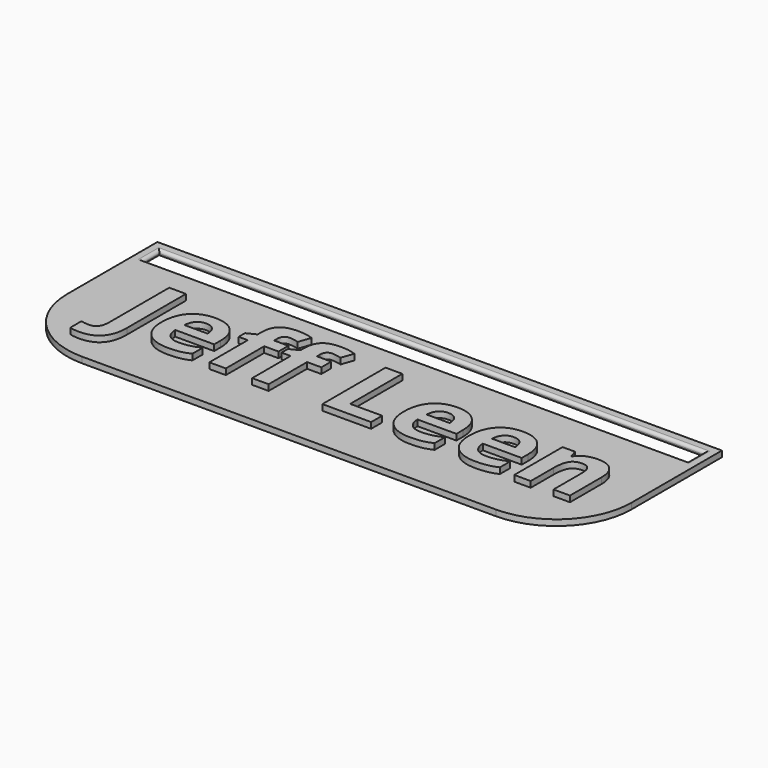
from build123d import *

# Parameters (mm, degrees)
F0_W         = 190.5
F0_H         = 63.5
F1_DEPTH     = 2
F2_W         = 183.896
F2_H         = 7.62
F3_DEPTH     = 25.4
F4_R         = 0.99999
F5_R         = 0.99999
F6_R         = 25.4
F7_TEXT_SIZE = 37.3212771969
F8_DEPTH     = 2


# Not quite as in the source:
# - a fillet or chamfer is up to 0.001 mm smaller than in the source, because OpenCascade refuses the exact size
# - Text() gives the source's letters only with a copy of the font that has no kerning and outlines rounded to 1/6400 em; it was checked with that copy


with BuildPart() as f1:
    # F0 (on Top) → F1 (new body)
    with BuildSketch(Plane.XY):
        with Locations((1.791532172, 31.75)):
            Rectangle(F0_W, F0_H)
    extrude(amount=F1_DEPTH)

    # F2 (on face) → F3 (cut)
    with BuildSketch(Plane.XY.offset(2)):
        with Locations((1.791532172, 56.388)):
            Rectangle(F2_W, F2_H)
    extrude(amount=-F3_DEPTH, mode=Mode.SUBTRACT)

    # F4 (radius 1 in the source; OpenCascade refuses exactly that, so slightly less here)
    f4_edges = [f1.edges().sort_by_distance(p)[0] for p in [
        (1.791532, 60.198, 2),
        (1.791532, 60.198, 0),
    ]]
    fillet(f4_edges, radius=F4_R)

    # F5 (radius 1 in the source; OpenCascade refuses exactly that, so slightly less here)
    f5_edges = [f1.edges().sort_by_distance(p)[0] for p in [
        (93.739532, 56.388, 0),
        (93.739532, 56.388, 2),
        (-90.156468, 56.388, 2),
        (-90.156468, 56.388, 0),
    ]]
    fillet(f5_edges, radius=F5_R)

    # F6
    f6_edges = [f1.edges().sort_by_distance(p)[0] for p in [
        (97.041532, 0, 1),
        (-93.458468, 0, 1),
    ]]
    fillet(f6_edges, radius=F6_R)

    # F7 (on face) → F8 (join)
    with BuildSketch(Plane.XY.offset(2)):
        with Locations((-75.678467828, 15.4231828795)):
            Text('Jeff Leen', F7_TEXT_SIZE, font='Open Sans', font_style=FontStyle.BOLD, text_align=(TextAlign.LEFT, TextAlign.BOTTOM))
    extrude(amount=F8_DEPTH)


solid = f1.part
